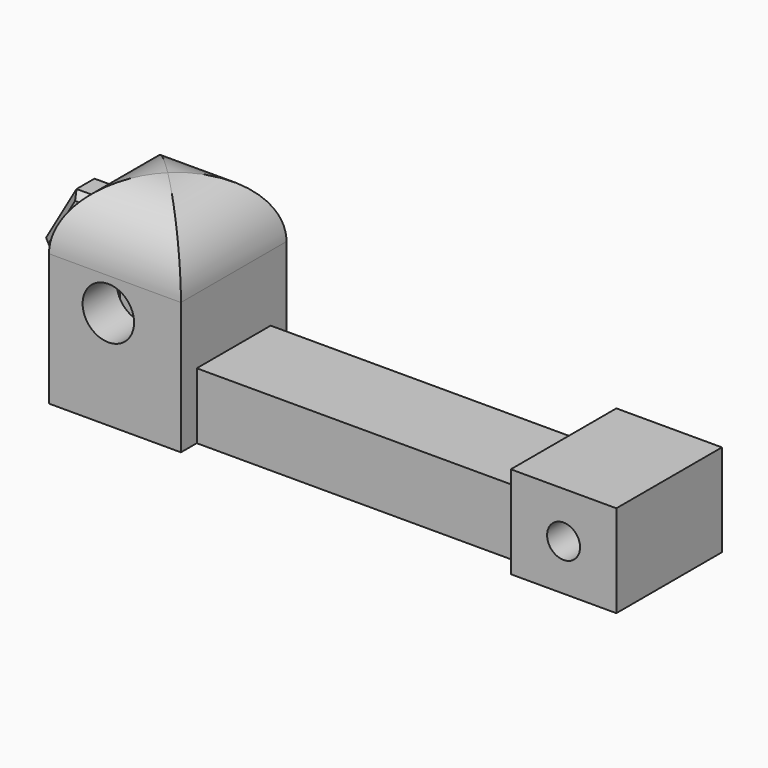
from build123d import *

# Parameters (mm, degrees)
F0_R        = 1.25
F1_DEPTH    = 10
F2_W        = 3.5
F2_H        = 8.5
F3_DEPTH    = 9
F4_R        = 1.95
F5_DEPTH    = 10
F6_T1_DEPTH = 35
F6_T3_DEPTH = 35
F7_W        = 25
F7_H        = 1.5
F8_DEPTH    = 5
F9_R        = 2
F10_DEPTH   = 2.7
F11_SIZE    = 0.5


# Not quite as in the source:
# - a fillet or chamfer that OpenCascade refuses, or shapes differently, is made with other operations: its cross-section is extruded or revolved along the edge and cut away or added


with BuildPart() as f1:
    # F0 (on Front) → F1 (new body)
    with BuildSketch(Plane.XZ):
        Polygon((10, 15), (0, 15), (0, 0), (43, 0), (43, 7), (35, 7), (35, 5), (10, 5), align=None)
        with Locations((39, 3.5)):
            Circle(F0_R, mode=Mode.SUBTRACT)
    extrude(amount=F1_DEPTH)

    # F2 (on face) → F3 (cut)
    with BuildSketch(Plane(origin=(0, 0, 0), x_dir=(0, -1, 0), z_dir=(-1, 0, 0))):
        with Locations((5, 7.5)):
            Rectangle(F2_W, F2_H)
    extrude(amount=-F3_DEPTH, mode=Mode.SUBTRACT)

    # F4 (on face) → F5 (cut, through all)
    with BuildSketch(Plane.XZ.offset(10)):
        with Locations((4.5, 7.5)):
            Circle(F4_R)
    extrude(amount=-F5_DEPTH, mode=Mode.SUBTRACT)

    # F6: fillet of radius 5 on 4 edges, made by hand

    # F6_s2 → F6_t1 (cut)
    with BuildSketch(Plane.XZ.offset(-12.5)):
        with BuildLine():
            ThreePointArc((5, 15), (8.5355339059, 13.5355339059), (10, 10))
            Line((10, 10), (10, 15))
            Line((10, 15), (5, 15))
        make_face()
        with BuildLine():
            ThreePointArc((5, 15), (1.4644660941, 13.5355339059), (0, 10))
            Line((0, 10), (0, 15))
            Line((0, 15), (5, 15))
        make_face()
    extrude(amount=F6_T1_DEPTH, mode=Mode.SUBTRACT)

    # F6_s4 → F6_t3 (cut)
    with BuildSketch(Plane.YZ.offset(-12.5)):
        with BuildLine():
            ThreePointArc((-5, 15), (-1.4644660941, 13.5355339059), (0, 10))
            Line((0, 10), (0, 15))
            Line((0, 15), (-5, 15))
        make_face()
        with BuildLine():
            ThreePointArc((-5, 15), (-8.5355339059, 13.5355339059), (-10, 10))
            Line((-10, 10), (-10, 15))
            Line((-10, 15), (-5, 15))
        make_face()
    extrude(amount=F6_T3_DEPTH, mode=Mode.SUBTRACT)

    # F7 (on face) → F8 (cut, through all)
    with BuildSketch(Plane.XY.offset(5)):
        with Locations((22.5, -0.75)):
            Rectangle(F7_W, F7_H)
        with Locations((22.5, -9.25)):
            Rectangle(F7_W, F7_H)
    extrude(amount=-F8_DEPTH, mode=Mode.SUBTRACT)


with BuildPart() as f10:
    # F9 (on Front) → F10 (new body)
    with BuildSketch(Plane.XZ):
        Polygon((-8.6188021535, 4), (-6.3094010768, 0), (-1.6905989232, 0), (0.6188021535, 4), (-1.6905989232, 8), (-6.3094010768, 8), align=None)
        with Locations((-4, 4)):
            Circle(F9_R, mode=Mode.SUBTRACT)
    extrude(amount=-F10_DEPTH)

    # F11
    f11_edges = [f10.edges().sort_by_distance(p)[0] for p in [
        (-7.464102, 2.7, 2),
        (-4, 2.7, 0),
        (-0.535898, 2.7, 2),
        (-0.535898, 2.7, 6),
        (-4, 2.7, 8),
        (-7.464102, 2.7, 6),
        (-6, 2.7, 4),
        (-7.464102, 0, 2),
        (-4, 0, 0),
        (-0.535898, 0, 2),
        (-0.535898, 0, 6),
        (-4, 0, 8),
        (-7.464102, 0, 6),
        (-6, 0, 4),
    ]]
    chamfer(f11_edges, length=F11_SIZE)


solid = Compound([f1.part, f10.part])
